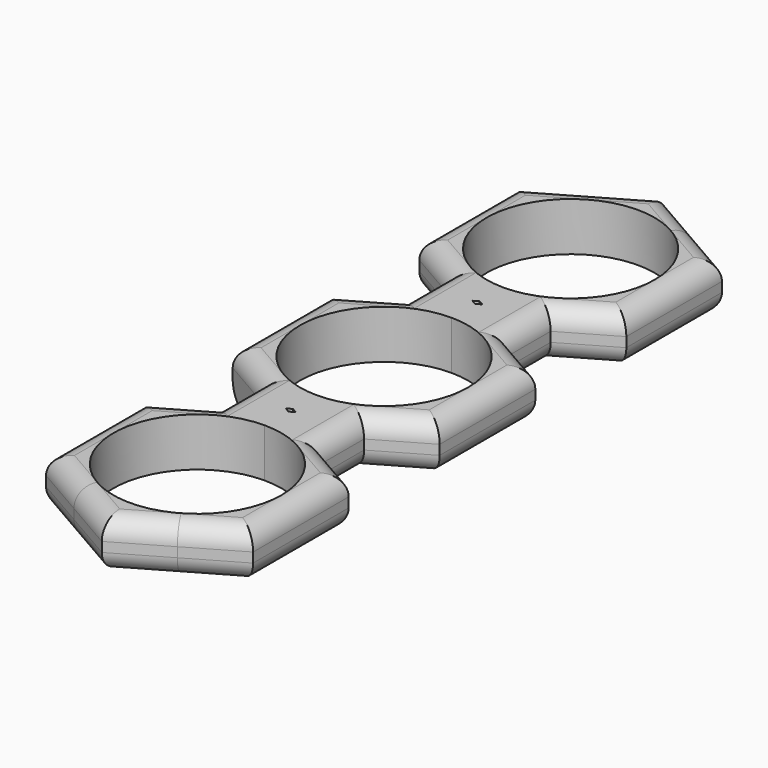
from build123d import *

# Parameters (mm, degrees)
F1_DEPTH = 6.35
F2_R     = 2.53999


# Not quite as in the source:
# - a fillet or chamfer is up to 0.001 mm smaller than in the source, because OpenCascade refuses the exact size


with BuildPart() as f1:
    # F0 (on Top) → F1 (new body)
    with BuildSketch(Plane.XY):
        with BuildLine():
            ThreePointArc((6.76275, -11.7134265989), (11.7134265989, -6.76275), (13.5255, 0))
            ThreePointArc((13.5255, 0), (11.7134265989, 6.76275), (6.76275, 11.7134265989))
            ThreePointArc((6.76275, 11.7134265989), (3.5006569945, 13.0646297635), (0, 13.5255))
            Line((0, 13.5255), (0, 10.9855))
            ThreePointArc((0, 10.9855), (7.7679215447, 7.7679215447), (10.9855, 0))
            ThreePointArc((10.9855, 0), (7.7679215447, -7.7679215447), (0, -10.9855))
            Line((0, -10.9855), (0, -13.5255))
            ThreePointArc((0, -13.5255), (3.5006569945, -13.0646297635), (6.76275, -11.7134265989))
        make_face()
        with BuildLine():
            Line((13.5255, -7.8089510659), (13.5255, 0))
            ThreePointArc((13.5255, 0), (11.7134265989, -6.76275), (6.76275, -11.7134265989))
            Line((6.76275, -11.7134265989), (13.5255, -7.8089510659))
        make_face()
        with BuildLine():
            ThreePointArc((6.76275, 11.7134265989), (11.7134265989, 6.76275), (13.5255, 0))
            Line((13.5255, 0), (13.5255, 7.8089510659))
            Line((13.5255, 7.8089510659), (6.76275, 11.7134265989))
        make_face()
        with BuildLine():
            ThreePointArc((0, 13.5255), (3.5006569945, 13.0646297635), (6.76275, 11.7134265989))
            Line((6.76275, 11.7134265989), (0.6545456927, 15.24))
            Line((0.6545456927, 15.24), (0, 14.8620978682))
            Line((0, 14.8620978682), (0, 13.5255))
        make_face()
        Polygon((0.6545456927, 15.24), (6.76275, 11.7134265989), (6.76275, 18.7665734011), align=None)
        with BuildLine():
            Line((0.6545456927, -15.24), (6.76275, -11.7134265989))
            ThreePointArc((6.76275, -11.7134265989), (3.5006569945, -13.0646297635), (0, -13.5255))
            Line((0, -13.5255), (0, -14.8620978682))
            Line((0, -14.8620978682), (0.6545456927, -15.24))
        make_face()
        Polygon((6.76275, -18.7665734011), (6.76275, -11.7134265989), (0.6545456927, -15.24), align=None)
        with BuildLine():
            Line((0, 10.9855), (0, 13.5255))
            ThreePointArc((0, 13.5255), (-3.5006569945, 13.0646297635), (-6.76275, 11.7134265989))
            ThreePointArc((-6.76275, 11.7134265989), (-11.7134265989, 6.76275), (-13.5255, 0))
            ThreePointArc((-13.5255, 0), (-11.7134265989, -6.76275), (-6.76275, -11.7134265989))
            ThreePointArc((-6.76275, -11.7134265989), (-3.5006569945, -13.0646297635), (0, -13.5255))
            Line((0, -13.5255), (0, -10.9855))
            ThreePointArc((0, -10.9855), (-10.9855, 0), (0, 10.9855))
        make_face()
        with BuildLine():
            ThreePointArc((-6.76275, 11.7134265989), (-3.5006569945, 13.0646297635), (0, 13.5255))
            Line((0, 13.5255), (0, 14.8620978682))
            Line((0, 14.8620978682), (-0.6545456927, 15.24))
            Line((-0.6545456927, 15.24), (-6.76275, 11.7134265989))
        make_face()
        with BuildLine():
            Line((0, 15.6179021318), (0.6545456927, 15.24))
            Line((0.6545456927, 15.24), (6.76275, 18.7665734011))
            ThreePointArc((6.76275, 18.7665734011), (3.5006569945, 17.4153702365), (0, 16.9545))
            Line((0, 16.9545), (0, 15.6179021318))
        make_face()
        with BuildLine():
            ThreePointArc((0, 16.9545), (3.5006569945, 17.4153702365), (6.76275, 18.7665734011))
            ThreePointArc((6.76275, 18.7665734011), (11.7134265989, 23.71725), (13.5255, 30.48))
            ThreePointArc((13.5255, 30.48), (11.7134266013, 37.2427499958), (6.7627500083, 42.1934265941))
            ThreePointArc((6.7627500083, 42.1934265941), (-1.056e-07, 44.0055), (-6.7627501912, 42.1934264885))
            ThreePointArc((-6.7627501912, 42.1934264885), (-11.7134266541, 37.2427499044), (-13.5255, 30.48))
            ThreePointArc((-13.5255, 30.48), (-11.7134265989, 23.71725), (-6.76275, 18.7665734011))
            ThreePointArc((-6.76275, 18.7665734011), (-3.5006569945, 17.4153702365), (0, 16.9545))
        make_face()
        with BuildLine():
            ThreePointArc((10.9855, 30.48), (7.7679215447, 22.7120784553), (0, 19.4945))
            ThreePointArc((0, 19.4945), (-7.7679215447, 38.2479215447), (10.9855, 30.48))
        make_face(mode=Mode.SUBTRACT)
        with BuildLine():
            ThreePointArc((13.5255, 30.48), (11.7134265989, 23.71725), (6.76275, 18.7665734011))
            Line((6.76275, 18.7665734011), (13.5255, 22.6710489341))
            Line((13.5255, 22.6710489341), (13.5255, 30.48))
        make_face()
        with BuildLine():
            Line((0, -14.8620978682), (0, -13.5255))
            ThreePointArc((0, -13.5255), (-3.5006569945, -13.0646297635), (-6.76275, -11.7134265989))
            Line((-6.76275, -11.7134265989), (-0.6545456927, -15.24))
            Line((-0.6545456927, -15.24), (0, -14.8620978682))
        make_face()
        with BuildLine():
            Line((6.76275, -18.7665734011), (0.6545456927, -15.24))
            Line((0.6545456927, -15.24), (0, -15.6179021318))
            Line((0, -15.6179021318), (0, -16.9545))
            ThreePointArc((0, -16.9545), (3.5006569945, -17.4153702365), (6.76275, -18.7665734011))
        make_face()
        with BuildLine():
            Line((13.5255, -22.6710489341), (6.76275, -18.7665734011))
            ThreePointArc((6.76275, -18.7665734011), (11.7134265989, -23.71725), (13.5255, -30.48))
            Line((13.5255, -30.48), (13.5255, -22.6710489341))
        make_face()
        with BuildLine():
            ThreePointArc((13.5255, -30.48), (11.7134265989, -23.71725), (6.76275, -18.7665734011))
            ThreePointArc((6.76275, -18.7665734011), (3.5006569945, -17.4153702365), (0, -16.9545))
            ThreePointArc((0, -16.9545), (-3.5006569945, -17.4153702365), (-6.76275, -18.7665734011))
            ThreePointArc((-6.76275, -18.7665734011), (-11.7134265989, -23.71725), (-13.5255, -30.48))
            ThreePointArc((-13.5255, -30.48), (-11.7134266419, -37.2427499255), (-6.762750149, -42.1934265129))
            ThreePointArc((-6.762750149, -42.1934265129), (-1.97e-07, -44.0055), (6.7627498078, -42.1934267099))
            ThreePointArc((6.7627498078, -42.1934267099), (11.7134265434, -37.2427500961), (13.5255, -30.48))
        make_face()
        with BuildLine():
            ThreePointArc((10.9855, -30.48), (-7.7679215447, -38.2479215447), (0, -19.4945))
            ThreePointArc((0, -19.4945), (7.7679215447, -22.7120784553), (10.9855, -30.48))
        make_face(mode=Mode.SUBTRACT)
        with BuildLine():
            ThreePointArc((-13.5255, 0), (-11.7134265989, 6.76275), (-6.76275, 11.7134265989))
            Line((-6.76275, 11.7134265989), (-13.5255, 7.8089510659))
            Line((-13.5255, 7.8089510659), (-13.5255, 0))
        make_face()
        Polygon((-6.76275, 18.7665734011), (-6.76275, 11.7134265989), (-0.6545456927, 15.24), align=None)
        with BuildLine():
            Line((-0.6545456927, 15.24), (0, 15.6179021318))
            Line((0, 15.6179021318), (0, 16.9545))
            ThreePointArc((0, 16.9545), (-3.5006569945, 17.4153702365), (-6.76275, 18.7665734011))
            Line((-6.76275, 18.7665734011), (-0.6545456927, 15.24))
        make_face()
        with BuildLine():
            ThreePointArc((6.7627500083, 42.1934265941), (11.7134266013, 37.2427499958), (13.5255, 30.48))
            Line((13.5255, 30.48), (13.5255, 38.2889510659))
            Line((13.5255, 38.2889510659), (6.7627500083, 42.1934265941))
        make_face()
        with BuildLine():
            Line((-13.5255, -7.8089510659), (-6.76275, -11.7134265989))
            ThreePointArc((-6.76275, -11.7134265989), (-11.7134265989, -6.76275), (-13.5255, 0))
            Line((-13.5255, 0), (-13.5255, -7.8089510659))
        make_face()
        Polygon((-0.6545456927, -15.24), (-6.76275, -11.7134265989), (-6.76275, -18.7665734011), align=None)
        with BuildLine():
            Line((0, -16.9545), (0, -15.6179021318))
            Line((0, -15.6179021318), (-0.6545456927, -15.24))
            Line((-0.6545456927, -15.24), (-6.76275, -18.7665734011))
            ThreePointArc((-6.76275, -18.7665734011), (-3.5006569945, -17.4153702365), (0, -16.9545))
        make_face()
        with BuildLine():
            Line((13.5255, -38.2889510659), (13.5255, -30.48))
            ThreePointArc((13.5255, -30.48), (11.7134265434, -37.2427500961), (6.7627498078, -42.1934267099))
            Line((6.7627498078, -42.1934267099), (13.5255, -38.2889510659))
        make_face()
        with BuildLine():
            Line((-13.5255, 22.6710489341), (-6.76275, 18.7665734011))
            ThreePointArc((-6.76275, 18.7665734011), (-11.7134265989, 23.71725), (-13.5255, 30.48))
            Line((-13.5255, 30.48), (-13.5255, 22.6710489341))
        make_face()
        with BuildLine():
            ThreePointArc((-6.7627501912, 42.1934264885), (-1.056e-07, 44.0055), (6.7627500083, 42.1934265941))
            Line((6.7627500083, 42.1934265941), (0, 46.0979021318))
            Line((0, 46.0979021318), (-6.7627501912, 42.1934264885))
        make_face()
        with BuildLine():
            ThreePointArc((-13.5255, -30.48), (-11.7134265989, -23.71725), (-6.76275, -18.7665734011))
            Line((-6.76275, -18.7665734011), (-13.5255, -22.6710489341))
            Line((-13.5255, -22.6710489341), (-13.5255, -30.48))
        make_face()
        with BuildLine():
            Line((0, -46.0979021318), (6.7627498078, -42.1934267099))
            ThreePointArc((6.7627498078, -42.1934267099), (-1.97e-07, -44.0055), (-6.762750149, -42.1934265129))
            Line((-6.762750149, -42.1934265129), (0, -46.0979021318))
        make_face()
        with BuildLine():
            Line((-13.5255, 38.2889510659), (-13.5255, 30.48))
            ThreePointArc((-13.5255, 30.48), (-11.7134266541, 37.2427499044), (-6.7627501912, 42.1934264885))
            Line((-6.7627501912, 42.1934264885), (-13.5255, 38.2889510659))
        make_face()
        with BuildLine():
            ThreePointArc((-6.762750149, -42.1934265129), (-11.7134266419, -37.2427499255), (-13.5255, -30.48))
            Line((-13.5255, -30.48), (-13.5255, -38.2889510659))
            Line((-13.5255, -38.2889510659), (-6.762750149, -42.1934265129))
        make_face()
    extrude(amount=F1_DEPTH)

    # F2 (radius 2.54 in the source; OpenCascade refuses exactly that, so slightly less here)
    f2_edges = [f1.edges().sort_by_distance(p)[0] for p in [
        (-6.76275, -42.193427, 6.35),
        (6.76275, -42.193427, 6.35),
        (13.5255, -30.48, 6.35),
        (-13.5255, -30.48, 6.35),
        (-10.144125, -20.718811, 6.35),
        (-6.76275, -15.24, 6.35),
        (10.144125, -20.718811, 6.35),
        (6.76275, -15.24, 6.35),
        (-10.144125, -9.761189, 6.35),
        (-13.5255, 0, 6.35),
        (-10.144125, 9.761189, 6.35),
        (-6.76275, 15.24, 6.35),
        (-10.144125, 20.718811, 6.35),
        (-13.5255, 30.48, 6.35),
        (-6.76275, 42.193427, 6.35),
        (6.76275, 42.193427, 6.35),
        (13.5255, 30.48, 6.35),
        (6.76275, 15.24, 6.35),
        (10.144125, 20.718811, 6.35),
        (10.144125, 9.761189, 6.35),
        (10.144125, -9.761189, 6.35),
        (13.5255, 0, 6.35),
        (-13.5255, -30.48, 0),
        (-6.76275, -42.193427, 0),
        (6.76275, -42.193427, 0),
        (13.5255, -30.48, 0),
        (10.144125, -20.718811, 0),
        (6.76275, -15.24, 0),
        (-10.144125, -20.718811, 0),
        (-6.76275, -15.24, 0),
        (-13.5255, 0, 0),
        (-10.144125, 9.761189, 0),
        (-6.76275, 15.24, 0),
        (-13.5255, 30.48, 0),
        (-6.76275, 42.193427, 0),
        (6.76275, 42.193427, 0),
        (13.5255, 30.48, 0),
        (10.144125, 20.718811, 0),
        (6.76275, 15.24, 0),
        (10.144125, 9.761189, 0),
        (10.144125, -9.761189, 0),
        (13.5255, 0, 0),
        (-10.144125, 20.718811, 0),
    ]]
    fillet(f2_edges, radius=F2_R)


solid = f1.part
